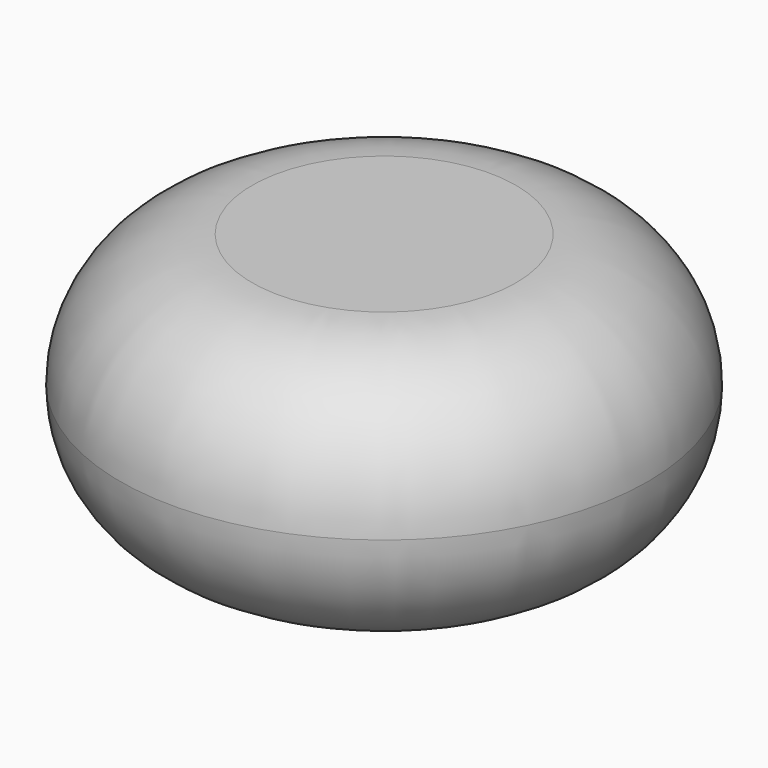
from build123d import *

# Parameters (mm, degrees)
F0_R     = 5
F1_DEPTH = 5
F2_R     = 2.49999


# Not quite as in the source:
# - a fillet or chamfer is up to 0.001 mm smaller than in the source, because OpenCascade refuses the exact size


with BuildPart() as f1:
    # F0 (on Top) → F1 (new body)
    with BuildSketch(Plane.XY):
        Circle(F0_R)
    extrude(amount=F1_DEPTH)

    # F2 (radius 2.5 in the source; OpenCascade refuses exactly that, so slightly less here)
    f2_edges = [f1.edges().sort_by_distance(p)[0] for p in [
        (-5, 0, 5),
        (-5, 0, 0),
    ]]
    fillet(f2_edges, radius=F2_R)


solid = f1.part
